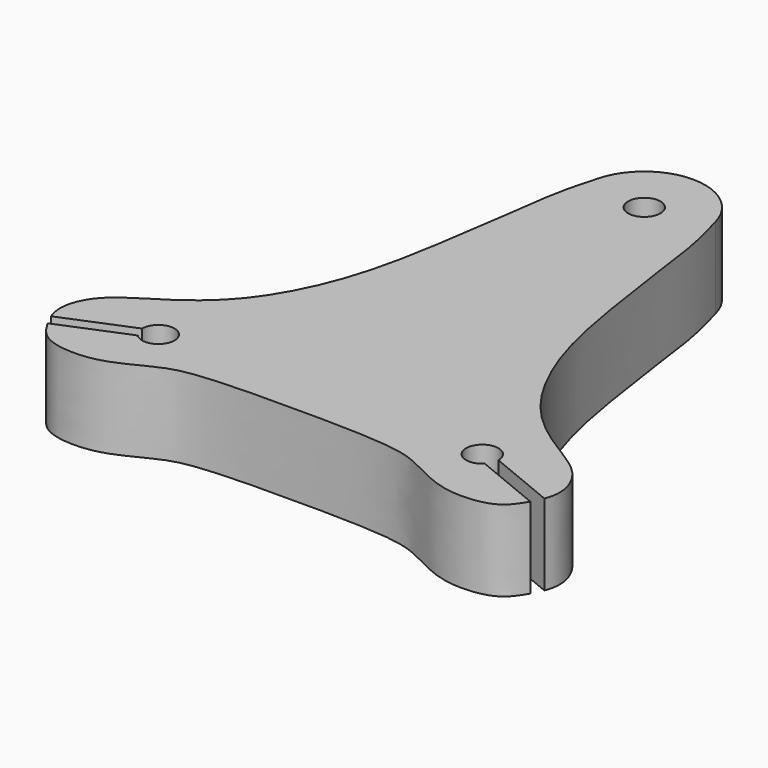
from build123d import *

# Parameters (mm, degrees)
F0_R     = 4
F1_DEPTH = 20


# Not quite as in the source:
# - a feature names something its author has since deleted; it is built from what else it names


with BuildPart() as f1:
    # F0 (on Top) → F1 (new body)
    with BuildSketch(Plane.XY):
        with BuildLine():
            add(Edge.make_bspline(
                [(14.5126224198, 60.7306027855), (16.8019810413, 52.9729625014), (17.9352869071, 44.6824925706), (21.4682283194, 18.795889632), (25.7689771102, -2.8067896835), (35.5622516207, -21.7126685978), (48.041945088, -31.286667461), (59.0700601288, -37.1336977452), (62.2848892569, -45.05003275), (61.3455249019, -48.9077577206), (60.9110098166, -50.047635349)],
                knots=[0, 0, 0, 0, 0.0835015327, 0.1819072556, 0.277438454, 0.367753358, 0.4463397859, 0.5157798719, 0.5748740106, 0.6017171757, 0.6017171757, 0.6017171757, 0.6017171757], degree=3))
            ThreePointArc((14.5126224198, 60.7306027855), (0, 71.9380059838), (-14.5126224198, 60.7306027855))
            add(Edge.make_bspline(
                [(-14.5126224198, 60.7306027855), (-16.8019810413, 52.9729625014), (-17.9352869071, 44.6824925706), (-21.4682283194, 18.795889632), (-25.7689771102, -2.8067896835), (-35.5622516207, -21.7126685978), (-48.041945088, -31.286667461), (-59.0700601288, -37.1336977452), (-62.2848892569, -45.05003275), (-61.3455249019, -48.9077577206), (-60.9110098166, -50.047635349)],
                knots=[0, 0, 0, 0, 0.0835015327, 0.1819072556, 0.277438454, 0.367753358, 0.4463397859, 0.5157798719, 0.5748740106, 0.6017171757, 0.6017171757, 0.6017171757, 0.6017171757], degree=3))
            Line((-60.9110098166, -50.047635349), (-43.9999255446, -43.0863997004))
            ThreePointArc((-43.9999255446, -43.0863997004), (-36.30112191, -41.5393972621), (-42.8579779791, -45.8605582679))
            Line((-42.8579779791, -45.8605582679), (-59.6026177667, -52.753279133))
            add(Edge.make_bspline(
                [(-59.6026177667, -52.753279133), (-59.5135605178, -52.9091652101), (-58.3731115182, -54.8631475989), (-55.9334692098, -58.202160494), (-48.5097440275, -59.5987131413), (-40.8258914603, -58.598927537), (-32.7700485865, -54.2100123222), (-25.276293749, -51.041569904), (-9.563678396, -50.8815310895), (0, -50.8815310895)],
                knots=[0.6240854269, 0.6240854269, 0.6240854269, 0.6240854269, 0.6281821208, 0.6760341184, 0.7287488094, 0.7845697385, 0.8433145605, 0.8993091345, 1, 1, 1, 1], degree=3))
            add(Edge.make_bspline(
                [(59.6026177667, -52.753279133), (59.5135605178, -52.9091652101), (58.3731115182, -54.8631475989), (55.9334692098, -58.202160494), (48.5097440275, -59.5987131413), (40.8258914603, -58.598927537), (32.7700485865, -54.2100123222), (25.276293749, -51.041569904), (9.563678396, -50.8815310895), (0, -50.8815310895)],
                knots=[0.6240854269, 0.6240854269, 0.6240854269, 0.6240854269, 0.6281821208, 0.6760341184, 0.7287488094, 0.7845697385, 0.8433145605, 0.8993091345, 1, 1, 1, 1], degree=3))
            Line((59.6026177667, -52.753279133), (42.8579779791, -45.8605582679))
            ThreePointArc((42.8579779791, -45.8605582679), (36.30112191, -41.5393972621), (43.9999255446, -43.0863997004))
            Line((43.9999255446, -43.0863997004), (60.9110098166, -50.047635349))
        make_face()
        with Locations((0, 56.9380059838)):
            Circle(F0_R, mode=Mode.SUBTRACT)
    extrude(amount=F1_DEPTH)


solid = f1.part
